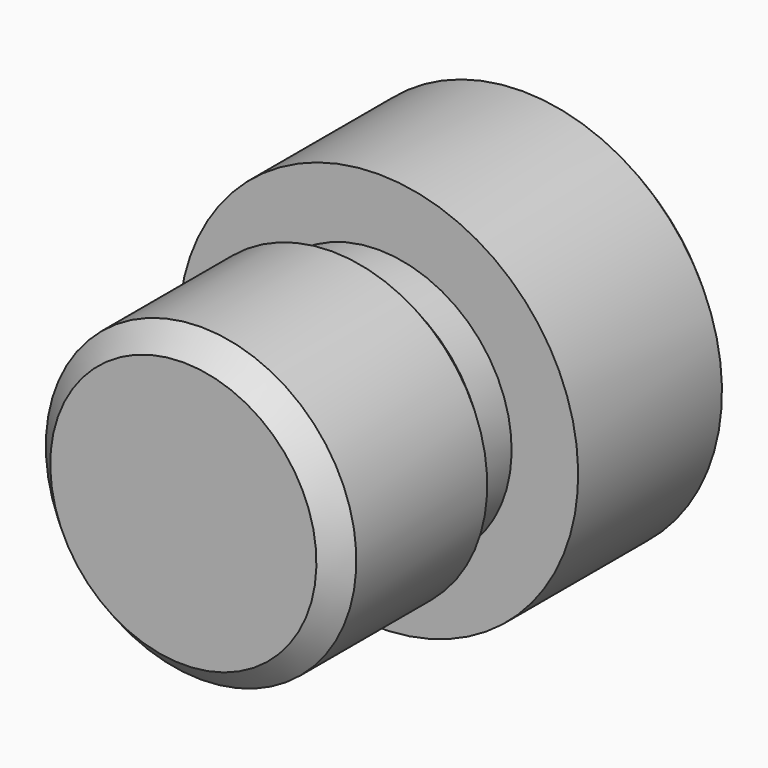
from build123d import *

# Parameters (mm, degrees)
F0_W    = 1.6225828454
F0_H    = 6
F2_SIZE = 0.99999


# Not quite as in the source:
# - a fillet or chamfer is up to 0.001 mm smaller than in the source, because OpenCascade refuses the exact size


with BuildPart() as f1:
    # F0 (on Right) → F1 (revolve)
    with BuildSketch(Plane.YZ):
        Polygon((11, 6), (11, 0), (19.1040290039, 0), (19.1040290039, 9), (11, 9), (11, 7), align=None)
        with BuildLine():
            Line((19.1040290039, 9), (19.1040290039, 0))
            Line((19.1040290039, 0), (23, 0))
            ThreePointArc((23, 0), (21.9842102668, 4.9035341847), (19.1040290039, 9))
        make_face()
        Polygon((0, 7), (0, 0), (9.3774171546, 0), (9.3774171546, 6), (9.3774171546, 7), align=None)
        with Locations((10.1887085773, 3)):
            Rectangle(F0_W, F0_H)
    revolve(axis=Axis((0, 9.5520145019, 0), (0, 1, 0)))

    # F2 (size 1 in the source; OpenCascade refuses exactly that, so slightly less here)
    f2_edges = [f1.edges().sort_by_distance(p)[0] for p in [
        (0, 9.377417, -7),
        (0, 0, -7),
    ]]
    chamfer(f2_edges, length=F2_SIZE)


solid = f1.part
